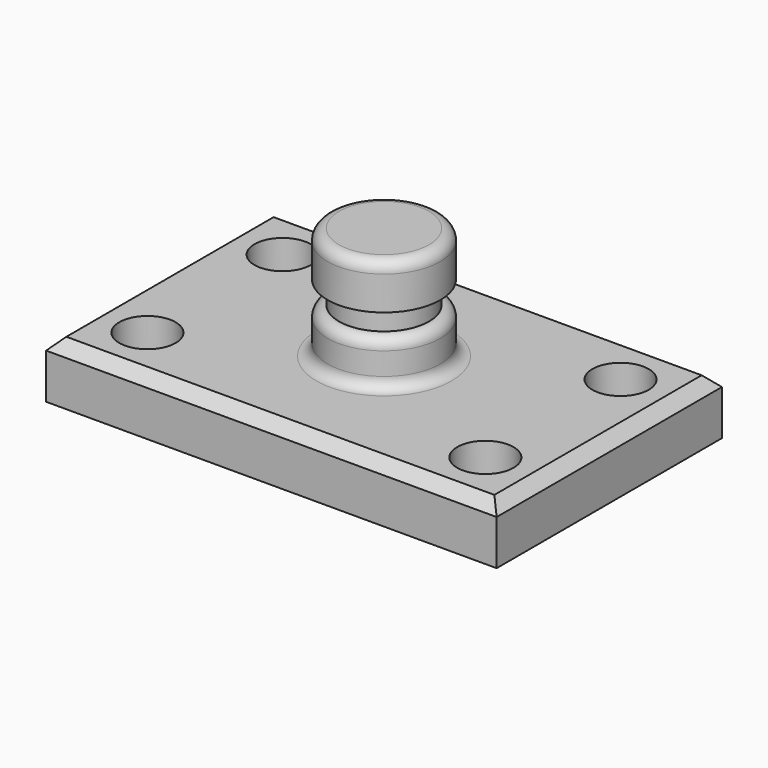
from build123d import *

# Parameters (mm, degrees)
F0_W     = 101.6
F0_H     = 63.5
F1_DEPTH = 12.7
F2_R     = 6.35
F3_DEPTH = 12.701
F4_W     = 12.7
F4_H     = 25.4
F6_W     = 4.7343277841
F6_H     = 5.08
F6_W_2   = 2.54
F8_R     = 2.53999
F9_R     = 2.54
F10_SIZE = 2.54


# Not quite as in the source:
# - a fillet or chamfer is up to 0.001 mm smaller than in the source, because OpenCascade refuses the exact size


with BuildPart() as f1:
    # F0 (on Top) → F1 (new body)
    with BuildSketch(Plane.XY):
        Rectangle(F0_W, F0_H)
    extrude(amount=F1_DEPTH)

    # F2 (on face) → F3 (cut, through all)
    with BuildSketch(Plane.XY.offset(12.7)):
        with Locations((-38.1, 19.05)):
            Circle(F2_R)
        with Locations((38.1, 19.05)):
            Circle(F2_R)
        with Locations((38.1, -19.05)):
            Circle(F2_R)
        with Locations((-38.1, -19.05)):
            Circle(F2_R)
    extrude(amount=-F3_DEPTH, mode=Mode.SUBTRACT)

    # F4 (on Front) → F5 (revolve)
    with BuildSketch(Plane.XZ):
        with Locations((6.35, 25.4)):
            Rectangle(F4_W, F4_H)
    revolve(axis=Axis((0, 0, 25.4), (0, 0, 1)))

    # F6 (on Front) → F7 (revolve, cut)
    with BuildSketch(Plane.XZ):
        with Locations((15.067163892, 25.4)):
            Rectangle(F6_W, F6_H)
        with Locations((11.43, 25.4)):
            Rectangle(F6_W_2, F6_H)
    revolve(axis=Axis((0, 0, 12.7), (0, 0, 1)), mode=Mode.SUBTRACT)

    # F8 (radius 2.54 in the source; OpenCascade refuses exactly that, so slightly less here)
    f8_edges = [f1.edges().sort_by_distance(p)[0] for p in [
        (-12.7, 0, 12.7),
        (-12.7, 0, 22.86),
    ]]
    fillet(f8_edges, radius=F8_R)

    # F9
    f9_edges = [f1.edges().sort_by_distance(p)[0] for p in [
        (-12.7, 0, 38.1),
    ]]
    fillet(f9_edges, radius=F9_R)

    # F10
    f10_edges = [f1.edges().sort_by_distance(p)[0] for p in [
        (-50.8, 0, 12.7),
        (0, -31.75, 12.7),
        (0, 31.75, 12.7),
        (50.8, 0, 12.7),
    ]]
    chamfer(f10_edges, length=F10_SIZE)


solid = f1.part
